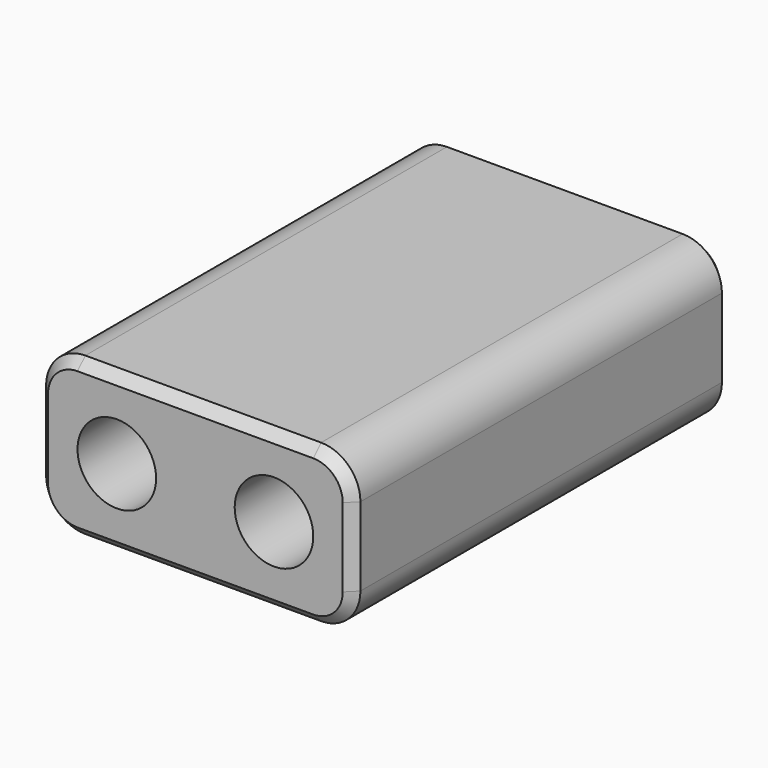
from build123d import *

# Parameters (mm, degrees)
F0_W     = 16
F0_H     = 24
F1_DEPTH = 8
F2_R     = 2
F3_DEPTH = 50
F5_R     = 2
F6_SIZE  = 0.5
F7_SIZE  = 1
F8_R     = 0.5


with BuildPart() as f1:
    # F0 (on Top) → F1 (new body)
    with BuildSketch(Plane.XY):
        Rectangle(F0_W, F0_H)
    extrude(amount=F1_DEPTH)

    # F2 (on face) → F3 (cut)
    with BuildSketch(Plane.XZ.offset(12)):
        with Locations((-4, 4)):
            Circle(F2_R)
    extrude(amount=-F3_DEPTH, mode=Mode.SUBTRACT)

    # F4: F1 across plane


with BuildPart() as f1_1:
    add(f1.part)
    add(f1.part.mirror(Plane.YZ), mode=Mode.INTERSECT)

    # F5
    f5_edges = [f1_1.edges().sort_by_distance(p)[0] for p in [
        (-8, 0, 8),
        (8, 0, 8),
        (8, 0, 0),
        (-8, 0, 0),
    ]]
    fillet(f5_edges, radius=F5_R)

    # F6
    f6_edges = [f1_1.edges().sort_by_distance(p)[0] for p in [
        (0, -12, 8),
        (0, 12, 8),
        (8, 12, 4),
        (7.414214, 12, 0.585786),
        (7.414214, 12, 7.414214),
        (0, 12, 0),
        (-7.414214, 12, 0.585786),
        (-7.414214, 12, 7.414214),
        (-8, 12, 4),
        (8, -12, 4),
        (7.414214, -12, 0.585786),
        (7.414214, -12, 7.414214),
        (0, -12, 0),
        (-7.414214, -12, 0.585786),
        (-7.414214, -12, 7.414214),
        (-8, -12, 4),
    ]]
    chamfer(f6_edges, length=F6_SIZE)

    # F7
    f7_edges = [f1_1.edges().sort_by_distance(p)[0] for p in [
        (6, 12, 4),
        (-6, 12, 4),
    ]]
    chamfer(f7_edges, length=F7_SIZE)

    # F8
    f8_edges = [f1_1.edges().sort_by_distance(p)[0] for p in [
        (-7, 12, 4),
        (7, 12, 4),
    ]]
    fillet(f8_edges, radius=F8_R)


solid = f1_1.part
